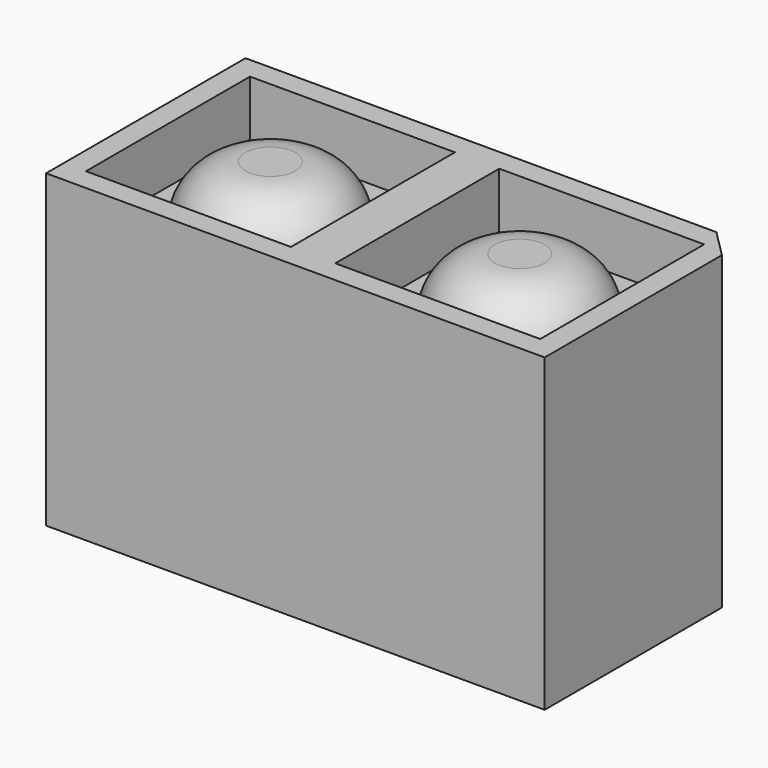
from build123d import *

# Parameters (mm, degrees)
F0_W     = 9
F0_H     = 4.5
F1_DEPTH = 5.6
F2_W     = 3.7
F2_H     = 3.7
F2_R     = 1.45
F3_DEPTH = 1
F4_R     = 0.99999
F5_SIZE  = 0.5


# Not quite as in the source:
# - a fillet or chamfer is up to 0.001 mm smaller than in the source, because OpenCascade refuses the exact size


with BuildPart() as f1:
    # F0 (on Top) → F1 (new body)
    with BuildSketch(Plane.XY):
        Rectangle(F0_W, F0_H)
    extrude(amount=F1_DEPTH)

    # F2 (on face) → F3 (cut)
    with BuildSketch(Plane.XY.offset(5.6)):
        with Locations((-2.25, 0)):
            Rectangle(F2_W, F2_H)
        with Locations((-2.25, 0)):
            Circle(F2_R, mode=Mode.SUBTRACT)
        with Locations((2.25, 0)):
            Rectangle(F2_W, F2_H)
        with Locations((2.25, 0)):
            Circle(F2_R, mode=Mode.SUBTRACT)
    extrude(amount=-F3_DEPTH, mode=Mode.SUBTRACT)

    # F4 (radius 1 in the source; OpenCascade refuses exactly that, so slightly less here)
    f4_edges = [f1.edges().sort_by_distance(p)[0] for p in [
        (-3.7, 0, 5.6),
        (0.8, 0, 5.6),
    ]]
    fillet(f4_edges, radius=F4_R)

    # F5
    f5_edges = [f1.edges().sort_by_distance(p)[0] for p in [
        (4.5, 2.25, 2.8),
    ]]
    chamfer(f5_edges, length=F5_SIZE)


solid = f1.part
